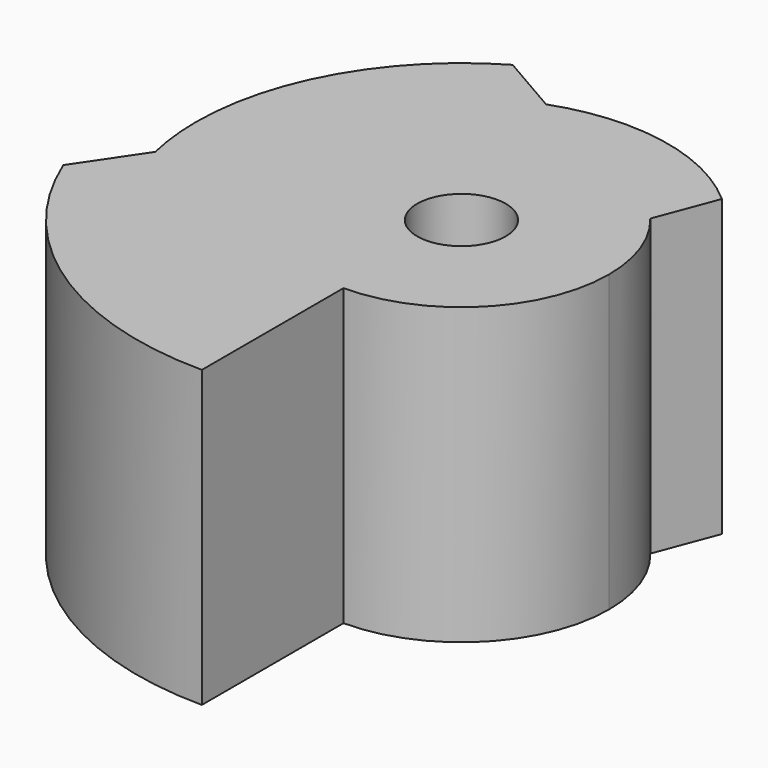
from build123d import *

# Parameters (mm, degrees)
F0_R         = 11
F0_R_2       = 1.5
F1_DEPTH     = 10
F3_DEPTH     = 25
F4_T4_DEPTH  = 31.4403610405
F4_S5_R      = 9
F4_T6_DEPTH  = 17
F4_T10_DEPTH = 33.7217724143
F4_S11_R     = 7
F4_T12_DEPTH = 19
F4_T16_DEPTH = 39.2279914145
F4_S17_R     = 5
F4_T18_DEPTH = 21


# Not quite as in the source:
# - a fillet or chamfer that OpenCascade refuses, or shapes differently, is made with other operations: its cross-section is extruded or revolved along the edge and cut away or added


with BuildPart() as f1:
    # F0 (on Top) → F1 (new body)
    with BuildSketch(Plane.XY):
        Circle(F0_R)
        Circle(F0_R_2, mode=Mode.SUBTRACT)
    extrude(amount=F1_DEPTH)

    # F2 (on face) → F3 (cut)
    with BuildSketch(Plane(origin=(0, 0, 0), x_dir=(1, 0, 0), z_dir=(0, 0, -1))):
        with BuildLine():
            ThreePointArc((0, -9), (-6.3639610307, -6.3639610307), (-9, 0))
            Line((-9, 0), (-11, 0))
            ThreePointArc((-11, 0), (-7.7781745931, -7.7781745931), (0, -11))
            Line((0, -11), (0, -9))
        make_face()
        with BuildLine():
            Line((11, 0), (9, 0))
            ThreePointArc((9, 0), (6.3639610307, -6.3639610307), (0, -9))
            Line((0, -9), (0, -11))
            ThreePointArc((0, -11), (7.7781745931, -7.7781745931), (11, 0))
        make_face()
        with BuildLine():
            Line((9, 0), (7, 0))
            ThreePointArc((7, 0), (4.9497474683, -4.9497474683), (0, -7))
            Line((0, -7), (0, -9))
            ThreePointArc((0, -9), (6.3639610307, -6.3639610307), (9, 0))
        make_face()
        with BuildLine():
            Line((0, 7), (0, 5))
            ThreePointArc((0, 5), (3.5355339059, 3.5355339059), (5, 0))
            Line((5, 0), (7, 0))
            ThreePointArc((7, 0), (4.9497474683, 4.9497474683), (0, 7))
        make_face()
        with BuildLine():
            Line((0, 9), (0, 7))
            ThreePointArc((0, 7), (4.9497474683, 4.9497474683), (7, 0))
            Line((7, 0), (9, 0))
            ThreePointArc((9, 0), (6.3639610307, 6.3639610307), (0, 9))
        make_face()
        with BuildLine():
            Line((0, 11), (0, 9))
            ThreePointArc((0, 9), (6.3639610307, 6.3639610307), (9, 0))
            Line((9, 0), (11, 0))
            ThreePointArc((11, 0), (7.7781745931, 7.7781745931), (0, 11))
        make_face()
    extrude(amount=-F3_DEPTH, mode=Mode.SUBTRACT)

    # F4: chamfer of 3 on 3 edges, made by hand


with BuildPart() as f4_tool2:
    # F4_s3 → F4_t4 (new body)
    with BuildSketch(Plane.XY.offset(-10.7201805202)):
        with BuildLine():
            Line((-10.1972729198, -4.125), (-7.4161984871, 0))
            Line((-7.4161984871, 0), (-11, 0))
            ThreePointArc((-11, 0), (-10.7891469286, -2.1434338231), (-10.1972729198, -4.125))
        make_face()
    extrude(amount=F4_T4_DEPTH)

    # F4_s5 → F4_t6 (cut, symmetric)
    with BuildSketch(Plane.XY.offset(5)):
        Circle(F4_S5_R)
    extrude(amount=F4_T6_DEPTH, both=True, mode=Mode.SUBTRACT)


with BuildPart() as f1_1:
    add(f1.part)

    # F4_t1: cut F4_tool2
    add(f4_tool2.part, mode=Mode.SUBTRACT)


with BuildPart() as f4_tool8:
    # F4_s9 → F4_t10 (new body)
    with BuildSketch(Plane.XY.offset(-11.8608862072)):
        with BuildLine():
            Line((-4.5, 7.7942286341), (0, 5.1961524227))
            Line((0, 5.1961524227), (0, 9))
            ThreePointArc((0, 9), (-2.3715637944, 8.6819171367), (-4.5, 7.7942286341))
        make_face()
    extrude(amount=F4_T10_DEPTH)

    # F4_s11 → F4_t12 (cut, symmetric)
    with BuildSketch(Plane.XY.offset(5)):
        Circle(F4_S11_R)
    extrude(amount=F4_T12_DEPTH, both=True, mode=Mode.SUBTRACT)


with BuildPart() as f1_2:
    add(f1_1.part)

    # F4_t7: cut F4_tool8
    add(f4_tool8.part, mode=Mode.SUBTRACT)


with BuildPart() as f4_tool14:
    # F4_s15 → F4_t16 (new body)
    with BuildSketch(Plane.XY.offset(-14.6139957073)):
        with BuildLine():
            Line((4.6300647944, 5.25), (2.6457513111, 0))
            Line((2.6457513111, 0), (7, 0))
            ThreePointArc((7, 0), (6.3609005548, 2.9221471784), (4.6300647944, 5.25))
        make_face()
    extrude(amount=F4_T16_DEPTH)

    # F4_s17 → F4_t18 (cut, symmetric)
    with BuildSketch(Plane.XY.offset(5)):
        Circle(F4_S17_R)
    extrude(amount=F4_T18_DEPTH, both=True, mode=Mode.SUBTRACT)


with BuildPart() as f1_3:
    add(f1_2.part)

    # F4_t13: cut F4_tool14
    add(f4_tool14.part, mode=Mode.SUBTRACT)


solid = f1_3.part
